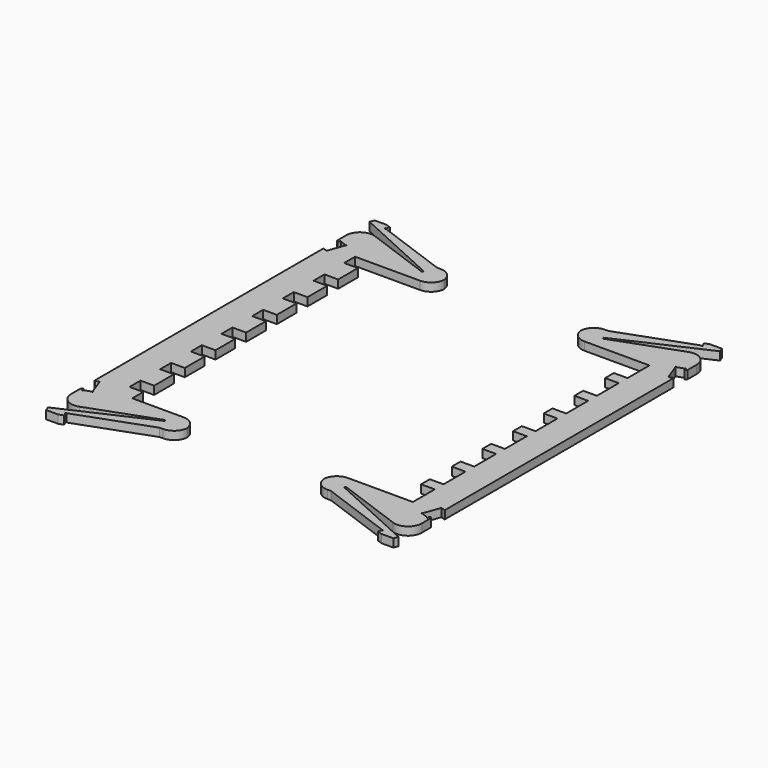
from build123d import *

# Parameters (mm, degrees)
F1_DEPTH        = 1.5
F4_W            = 5
F4_H            = 10
F5_DEPTH        = 3
F6_W            = 23.75
F6_H            = 108
F6_W_2          = 50
F6_H_2          = 26
F7_DEPTH        = 3
F8_W            = 5
F8_H            = 5
F9_DEPTH        = 3
F10_T1_DEPTH    = 38.7037001686
F10_T3_DEPTH    = 28
F10_S1_T1_DEPTH = 38.7037001686
F10_S1_T3_DEPTH = 28


# Not quite as in the source:
# - a fillet or chamfer that OpenCascade refuses, or shapes differently, is made with other operations: its cross-section is extruded or revolved along the edge and cut away or added
# - a feature names something its author has since deleted; it is built from what else it names


with BuildPart() as f1:
    # F0 (on Top) → F1 (new body, symmetric)
    with BuildSketch(Plane.XY):
        with BuildLine():
            Line((31.2800427974, 63.3035998776), (0, 63.3035998776))
            Line((0, 63.3035998776), (0, 0))
            Line((0, 0), (64, 0))
            Line((64, 0), (64, 52.0472386562))
            ThreePointArc((64, 52.0472386562), (63.9147152873, 52.211069065), (63.7315959713, 52.2351771803))
            Line((63.7315959713, 52.2351771803), (62.4040530693, 51.7519910793))
            Line((62.4040530693, 51.7519910793), (60.2493261663, 57.6720545902))
            ThreePointArc((60.2493261663, 57.6720545902), (59.9996605802, 57.9445167667), (60.3688606618, 57.9283971431))
            Line((60.3688606618, 57.9283971431), (62.8120614758, 58.8176495157))
            ThreePointArc((62.8120614758, 58.8176495157), (63.0845236523, 59.0673151018), (63.0684040287, 58.6981150202))
            Line((63.0684040287, 58.6981150202), (63.2443290661, 58.2147649522))
            ThreePointArc((63.2443290661, 58.2147649522), (63.3805037813, 58.0899838157), (63.5608251122, 58.1299600923))
            Line((63.5608251122, 58.1299600923), (63.9285575219, 58.4385242216))
            ThreePointArc((63.9285575219, 58.4385242216), (63.9812615574, 58.5072094579), (64, 58.5917331103))
            Line((64, 58.5917331103), (64, 69.8918015034))
            Line((64, 69.8918015034), (32.9901435141, 58.6051367736))
            Line((32.9901435141, 58.6051367736), (32.7849314281, 59.1689523461))
            Line((32.7849314281, 59.1689523461), (64, 73.3944786626))
            Line((64, 73.3944786626), (63.4156380227, 75))
            Line((63.4156380227, 75), (59.0299314225, 75))
            Line((59.0299314225, 75), (57.3566676351, 74.3909817873))
            Line((57.3566676351, 74.3909817873), (57.8012938214, 73.1693813803))
            ThreePointArc((57.8012938214, 73.1693813803), (58.0509594075, 72.8969192038), (57.681759326, 72.9130388275))
            Line((57.681759326, 72.9130388275), (31.2800427974, 63.3035998776))
        make_face()
    extrude(amount=F1_DEPTH, both=True)

    # F2: F1 across face


with BuildPart() as f1_1:
    add(f1.part)
    add(f1.part.mirror(Plane(origin=(0, 31.6517999388, 0), x_dir=(0, -1, 0), z_dir=(-1, 0, 0))))

    # F3: F1 across face


with BuildPart() as f1_2:
    add(f1_1.part)
    add(f1_1.part.mirror(Plane.XZ))

    # F4 (on face) → F5 (cut)
    with BuildSketch(Plane.XY.offset(1.5)):
        with Locations((-51.25, -49)):
            Rectangle(F4_W, F4_H)
        with Locations((-51.25, -35)):
            Rectangle(F4_W, F4_H)
        with Locations((-51.25, -21)):
            Rectangle(F4_W, F4_H)
        with Locations((-51.25, -7)):
            Rectangle(F4_W, F4_H)
        with Locations((-51.25, 7)):
            Rectangle(F4_W, F4_H)
        with Locations((-51.25, 21)):
            Rectangle(F4_W, F4_H)
        with Locations((-51.25, 35)):
            Rectangle(F4_W, F4_H)
        with Locations((51.25, -49)):
            Rectangle(F4_W, F4_H)
        with Locations((51.25, -35)):
            Rectangle(F4_W, F4_H)
        with Locations((51.25, -21)):
            Rectangle(F4_W, F4_H)
        with Locations((51.25, -7)):
            Rectangle(F4_W, F4_H)
        with Locations((51.25, 7)):
            Rectangle(F4_W, F4_H)
        with Locations((51.25, 21)):
            Rectangle(F4_W, F4_H)
        with Locations((51.25, 35)):
            Rectangle(F4_W, F4_H)
        with Locations((-51.25, 49)):
            Rectangle(F4_W, F4_H)
        with Locations((51.25, 49)):
            Rectangle(F4_W, F4_H)
    extrude(amount=-F5_DEPTH, mode=Mode.SUBTRACT)

    # F6 (on face) → F7 (cut)
    with BuildSketch(Plane.XY.offset(1.5)):
        with Locations((36.875, 0)):
            Rectangle(F6_W, F6_H)
        Rectangle(F6_W_2, F6_H)
        with Locations((0, 67)):
            Rectangle(F6_W_2, F6_H_2)
        with Locations((-36.875, 0)):
            Rectangle(F6_W, F6_H)
        with Locations((0, -67)):
            Rectangle(F6_W_2, F6_H_2)
    extrude(amount=-F7_DEPTH, mode=Mode.SUBTRACT)

    # F8 (on face) → F9 (join, through all)
    with BuildSketch(Plane.XY.offset(1.5)):
        with Locations((-51.25, -51.5)):
            Rectangle(F8_W, F8_H)
        with Locations((-51.25, -37.5)):
            Rectangle(F8_W, F8_H)
        with Locations((-51.25, -23.5)):
            Rectangle(F8_W, F8_H)
        with Locations((-51.25, -9.5)):
            Rectangle(F8_W, F8_H)
        with Locations((-51.25, 4.5)):
            Rectangle(F8_W, F8_H)
        with Locations((-51.25, 18.5)):
            Rectangle(F8_W, F8_H)
        with Locations((-51.25, 32.5)):
            Rectangle(F8_W, F8_H)
        with Locations((-51.25, 46.5)):
            Rectangle(F8_W, F8_H)
    extrude(amount=-F9_DEPTH)

    # F10: fillet of radius 5 on 6 edges, made by hand

    # F10_s2 → F10_t1 (cut)
    with BuildSketch(Plane.XY.offset(-19.3518500843)):
        with BuildLine():
            ThreePointArc((-64, 62.7510614697), (-61.8678821818, 66.8468216911), (-57.2898992834, 67.4495245736))
            Line((-57.2898992834, 67.4495245736), (-64, 69.8918015034))
            Line((-64, 69.8918015034), (-64, 62.7510614697))
        make_face()
        with BuildLine():
            ThreePointArc((-57.2898992834, -67.4495245736), (-61.8678821818, -66.8468216911), (-64, -62.7510614697))
            Line((-64, -62.7510614697), (-64, -69.8918015034))
            Line((-64, -69.8918015034), (-57.2898992834, -67.4495245736))
        make_face()
    extrude(amount=F10_T1_DEPTH, mode=Mode.SUBTRACT)

    # F10_s4 → F10_t3 (cut)
    with BuildSketch(Plane.XY.offset(-14)):
        with BuildLine():
            ThreePointArc((-30, 63.3035998776), (-26.4644660941, 61.8391337835), (-25, 58.3035998776))
            Line((-25, 58.3035998776), (-25, 63.3035998776))
            Line((-25, 63.3035998776), (-30, 63.3035998776))
        make_face()
        with BuildLine():
            ThreePointArc((-30, -54), (-26.4644660941, -55.4644660941), (-25, -59))
            Line((-25, -59), (-25, -54))
            Line((-25, -54), (-30, -54))
        make_face()
        with BuildLine():
            ThreePointArc((-30, 54), (-26.4644660941, 55.4644660941), (-25, 59))
            Line((-25, 59), (-25, 54))
            Line((-25, 54), (-30, 54))
        make_face()
        with BuildLine():
            ThreePointArc((-25, -58.3035998776), (-26.4644660941, -61.8391337835), (-30, -63.3035998776))
            Line((-30, -63.3035998776), (-25, -63.3035998776))
            Line((-25, -63.3035998776), (-25, -58.3035998776))
        make_face()
    extrude(amount=F10_T3_DEPTH, mode=Mode.SUBTRACT)

    # F10#s1: fillet of radius 5 on 6 edges, made by hand

    # F10_s1_s2 → F10_s1_t1 (cut)
    with BuildSketch(Plane.XY.offset(-19.3518500843)):
        with BuildLine():
            ThreePointArc((57.2898992834, 67.4495245736), (61.8678821818, 66.8468216911), (64, 62.7510614697))
            Line((64, 62.7510614697), (64, 69.8918015034))
            Line((64, 69.8918015034), (57.2898992834, 67.4495245736))
        make_face()
        with BuildLine():
            ThreePointArc((64, -62.7510614697), (61.8678821818, -66.8468216911), (57.2898992834, -67.4495245736))
            Line((57.2898992834, -67.4495245736), (64, -69.8918015034))
            Line((64, -69.8918015034), (64, -62.7510614697))
        make_face()
    extrude(amount=F10_S1_T1_DEPTH, mode=Mode.SUBTRACT)

    # F10_s1_s4 → F10_s1_t3 (cut)
    with BuildSketch(Plane.XY.offset(-14)):
        with BuildLine():
            ThreePointArc((25, 58.3035998776), (26.4644660941, 61.8391337835), (30, 63.3035998776))
            Line((30, 63.3035998776), (25, 63.3035998776))
            Line((25, 63.3035998776), (25, 58.3035998776))
        make_face()
        with BuildLine():
            ThreePointArc((30, 54), (26.4644660941, 55.4644660941), (25, 59))
            Line((25, 59), (25, 54))
            Line((25, 54), (30, 54))
        make_face()
        with BuildLine():
            ThreePointArc((25, -59), (26.4644660941, -55.4644660941), (30, -54))
            Line((30, -54), (25, -54))
            Line((25, -54), (25, -59))
        make_face()
        with BuildLine():
            ThreePointArc((30, -63.3035998776), (26.4644660941, -61.8391337835), (25, -58.3035998776))
            Line((25, -58.3035998776), (25, -63.3035998776))
            Line((25, -63.3035998776), (30, -63.3035998776))
        make_face()
    extrude(amount=F10_S1_T3_DEPTH, mode=Mode.SUBTRACT)


solid = f1_2.part
